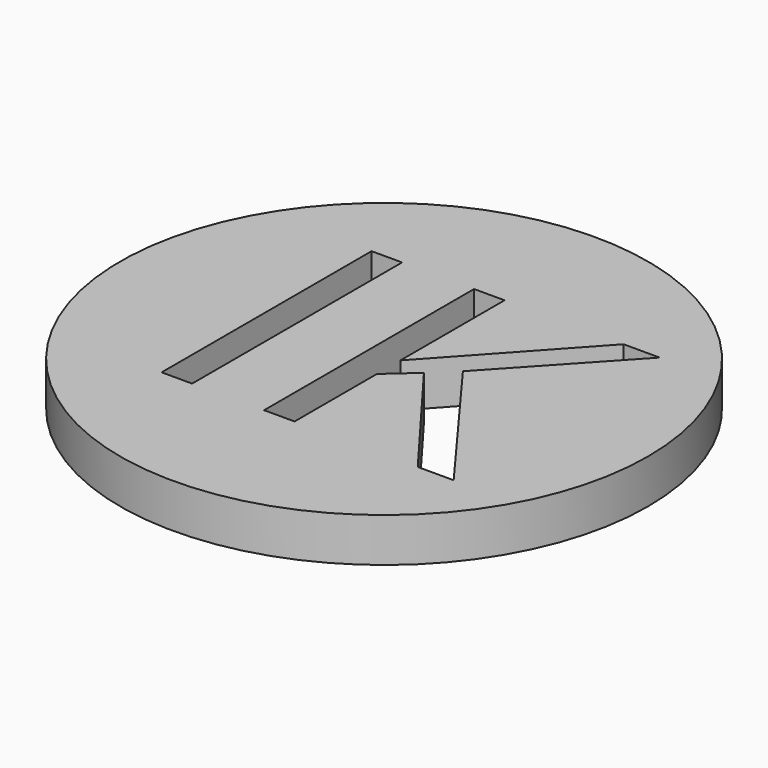
from build123d import *

# Parameters (mm, degrees)
F0_R         = 12
F1_DEPTH     = 2
F2_TEXT_SIZE = 16.7129100702
F3_DEPTH     = 25


# Not quite as in the source:
# - Text() gives the source's letters only with a copy of the font that has no kerning and outlines rounded to 1/6400 em; it was checked with that copy


with BuildPart() as f1:
    # F0 (on Top) → F1 (new body)
    with BuildSketch(Plane.XY):
        Circle(F0_R)
    extrude(amount=F1_DEPTH)

    # F2 (on face) → F3 (cut)
    with BuildSketch(Plane.XY.offset(2)):
        with Locations((-7.1651054116, -5.7360520969)):
            Text('IK', F2_TEXT_SIZE, font='Open Sans', text_align=(TextAlign.LEFT, TextAlign.BOTTOM))
    extrude(amount=-F3_DEPTH, mode=Mode.SUBTRACT)


solid = f1.part
